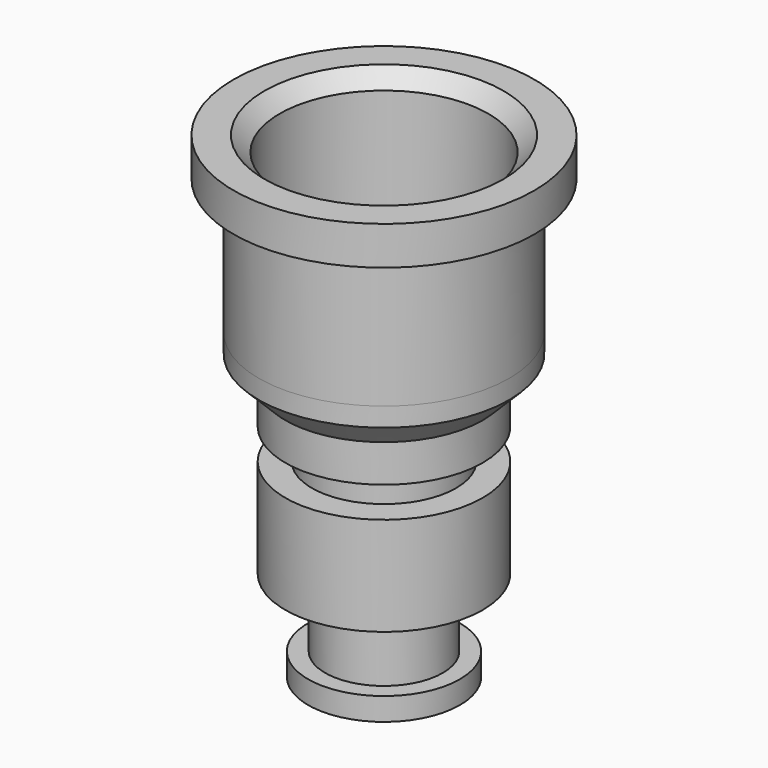
from build123d import *

# Parameters (mm, degrees)
F0_R      = 6.5
F0_R_2    = 2.75
F1_DEPTH  = 20
F2_R      = 6.5
F2_R_2    = 5
F3_DEPTH  = 6
F4_R      = 5
F4_R_2    = 3.875
F5_DEPTH  = 4.5
F7_R      = 6.5
F7_R_2    = 4.75
F8_DEPTH  = 2.032
F9_R      = 8.25
F9_R_2    = 6.5
F10_DEPTH = 3
F11_R     = 8.25
F11_R_2   = 6.875
F12_DEPTH = 11.43
F13_R     = 9.906
F13_R_2   = 8.25
F14_DEPTH = 2.54
F15_SIZE  = 1.74999
F16_SIZE  = 1
F17_SIZE  = 0.5
F18_SIZE  = 1


# Not quite as in the source:
# - a fillet or chamfer is up to 0.001 mm smaller than in the source, because OpenCascade refuses the exact size


with BuildPart() as f1:
    # F0 (on Top) → F1 (new body)
    with BuildSketch(Plane.XY):
        Circle(F0_R)
        Circle(F0_R_2, mode=Mode.SUBTRACT)
    extrude(amount=F1_DEPTH)

    # F2 (on face) → F3 (cut)
    with BuildSketch(Plane(origin=(0, 0, 0), x_dir=(1, 0, 0), z_dir=(0, 0, -1))):
        Circle(F2_R)
        Circle(F2_R_2, mode=Mode.SUBTRACT)
    extrude(amount=-F3_DEPTH, mode=Mode.SUBTRACT)

    # F4 (on face) → F5 (cut)
    with BuildSketch(Plane(origin=(0, 0, 6), x_dir=(1, 0, 0), z_dir=(0, 0, -1))):
        Circle(F4_R)
        Circle(F4_R_2, mode=Mode.SUBTRACT)
    extrude(amount=F5_DEPTH, mode=Mode.SUBTRACT)

    # F7 (on offset) → F8 (cut)
    with BuildSketch(Plane(origin=(0, 0, 12.5), x_dir=(1, 0, 0), z_dir=(0, 0, -1))):
        Circle(F7_R)
        Circle(F7_R_2, mode=Mode.SUBTRACT)
    extrude(amount=-F8_DEPTH, mode=Mode.SUBTRACT)

    # F9 (on face) → F10 (join)
    with BuildSketch(Plane.XY.offset(20)):
        Circle(F9_R)
        Circle(F9_R_2, mode=Mode.SUBTRACT)
    extrude(amount=-F10_DEPTH)

    # F11 (on face) → F12 (join)
    with BuildSketch(Plane.XY.offset(20)):
        Circle(F11_R)
        Circle(F11_R_2, mode=Mode.SUBTRACT)
    extrude(amount=F12_DEPTH)

    # F13 (on face) → F14 (join)
    with BuildSketch(Plane.XY.offset(31.43)):
        Circle(F13_R)
        Circle(F13_R_2, mode=Mode.SUBTRACT)
    extrude(amount=-F14_DEPTH)

    # F15 (size 1.75 in the source; OpenCascade refuses exactly that, so slightly less here)
    f15_edges = [f1.edges().sort_by_distance(p)[0] for p in [
        (-8.25, 0, 17),
    ]]
    chamfer(f15_edges, length=F15_SIZE)

    # F16
    f16_edges = [f1.edges().sort_by_distance(p)[0] for p in [
        (-6.875, 0, 31.43),
    ]]
    chamfer(f16_edges, length=F16_SIZE)

    # F17
    f17_edges = [f1.edges().sort_by_distance(p)[0] for p in [
        (-2.75, 0, 0),
    ]]
    chamfer(f17_edges, length=F17_SIZE)

    # F18
    f18_edges = [f1.edges().sort_by_distance(p)[0] for p in [
        (-2.75, 0, 20),
    ]]
    chamfer(f18_edges, length=F18_SIZE)


solid = f1.part
